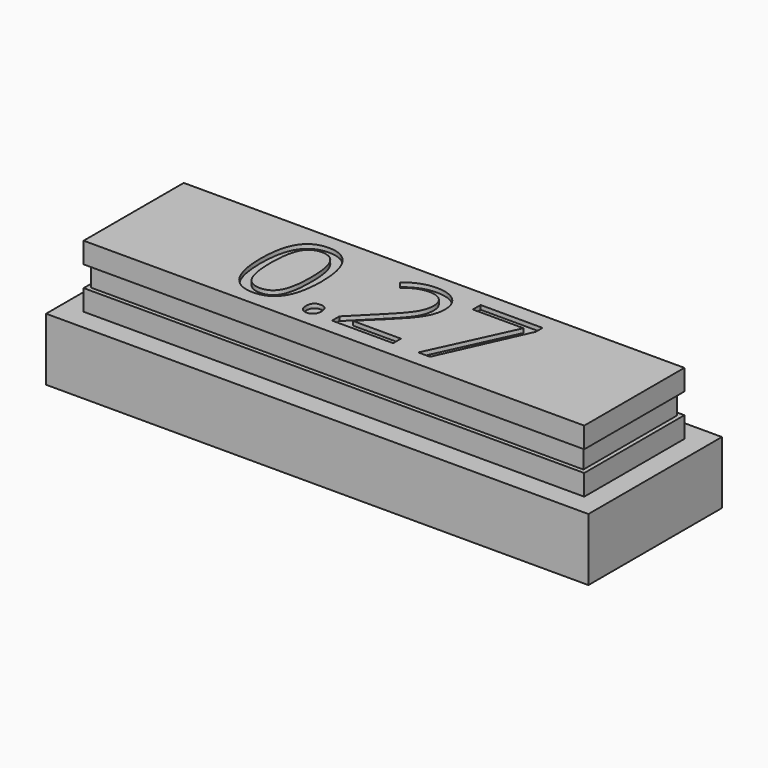
from build123d import *

# Parameters (mm, degrees)
F0_W         = 26
F0_H         = 8
F0_W_2       = 20
F0_H_2       = 2
F1_DEPTH     = 3
F2_W         = 24
F2_H         = 6
F3_DEPTH     = 3
F5_W         = 24
F5_H         = 6
F5_W_2       = 23.6
F5_H_2       = 5.6
F6_DEPTH     = 0.5
F7_W         = 19.46
F7_H         = 1.46
F8_DEPTH     = 3
F9_TEXT_SIZE = 6.25
F10_DEPTH    = 0.2


# Not quite as in the source:
# - Text() gives the source's letters only with a copy of the font that has no kerning and outlines rounded to 1/6400 em; it was checked with that copy


with BuildPart() as f1:
    # F0 (on Top) → F1 (new body)
    with BuildSketch(Plane.XY):
        Rectangle(F0_W, F0_H)
        Rectangle(F0_W_2, F0_H_2, mode=Mode.SUBTRACT)
    extrude(amount=F1_DEPTH)


with BuildPart() as f3:
    # F2 (on face) → F3 (new body)
    with BuildSketch(Plane.XY.offset(3)):
        Rectangle(F2_W, F2_H)
    extrude(amount=F3_DEPTH)

    # F5 (on mid) → F6 (cut, symmetric)
    with BuildSketch(Plane.XY.offset(4.5)):
        Rectangle(F5_W, F5_H)
        Rectangle(F5_W_2, F5_H_2, mode=Mode.SUBTRACT)
    extrude(amount=F6_DEPTH, both=True, mode=Mode.SUBTRACT)

    # F7 (on face) → F8 (join, through all)
    with BuildSketch(Plane(origin=(0, 0, 3), x_dir=(1, 0, 0), z_dir=(0, 0, -1))):
        Rectangle(F7_W, F7_H)
    extrude(amount=F8_DEPTH)

    # F9 (on face) → F10 (cut)
    with BuildSketch(Plane.XY.offset(6)):
        with Locations((-6.2353515625, -2.25)):
            Text('0.27', F9_TEXT_SIZE, font='Open Sans', text_align=(TextAlign.LEFT, TextAlign.BOTTOM))
    extrude(amount=-F10_DEPTH, mode=Mode.SUBTRACT)


solid = Compound([f1.part, f3.part])
